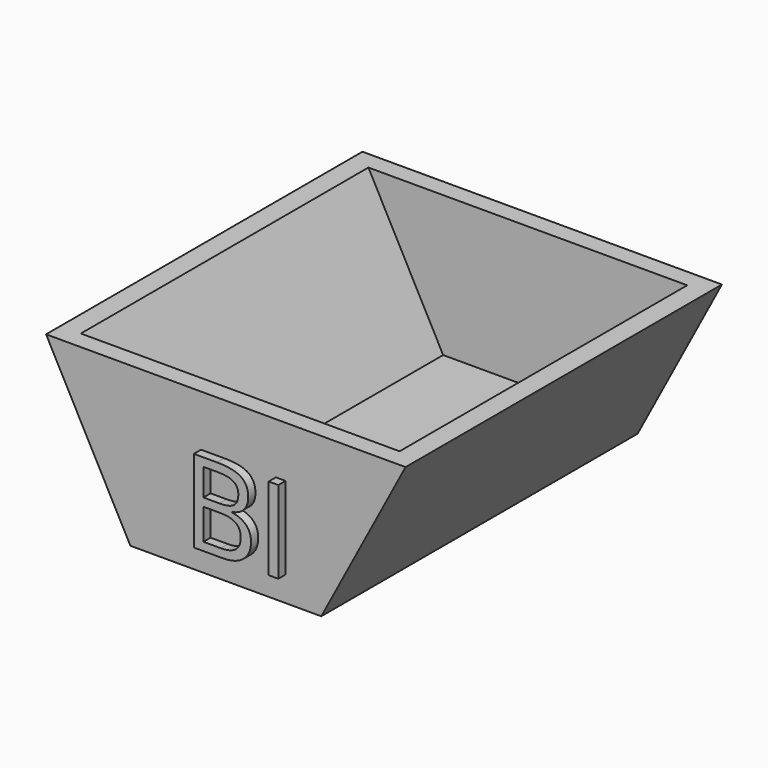
from build123d import *

# Parameters (mm, degrees)
F1_DEPTH     = 55.88
F2_T         = -2.54
F3_TEXT_SIZE = 16.3294374943
F4_DEPTH     = 1.27


# Not quite as in the source:
# - Text() gives the source's letters only with a copy of the font that has no kerning and outlines rounded to 1/6400 em; it was checked with that copy


with BuildPart() as f1:
    # F0 (on Front) → F1 (new body)
    with BuildSketch(Plane.XZ):
        Polygon((15.9106230548, 18.8914433397), (-34.8893769452, 18.8914433397), (-22.9779180269, -3.5423959758), (3.9991641364, -3.5423959758), align=None)
    extrude(amount=F1_DEPTH)

    # F2
    f2_openings = [f1.faces().sort_by_distance(p)[0] for p in [
        (-9.489377, -27.94, 18.891443),
    ]]
    offset(amount=F2_T, openings=f2_openings)

    # F3 (on face) → F4 (join)
    with BuildSketch(Plane.XZ.offset(55.88)):
        with Locations((-14.5969862351, 0)):
            Text('BI', F3_TEXT_SIZE, font='Open Sans', text_align=(TextAlign.LEFT, TextAlign.BOTTOM))
    extrude(amount=F4_DEPTH)


solid = f1.part
